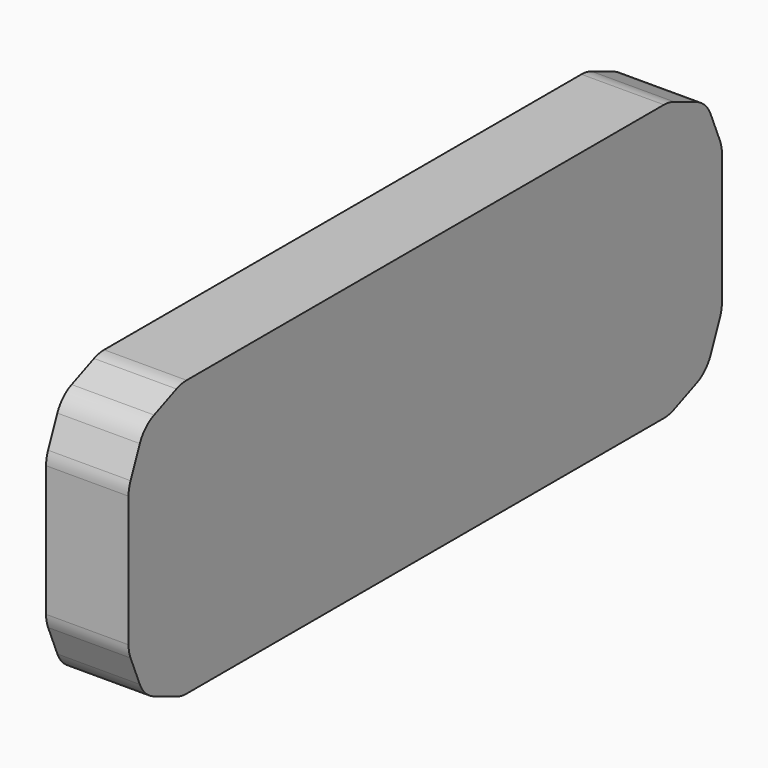
from build123d import *

# Parameters (mm, degrees)
F0_W        = 114.2217256129
F0_H        = 42.490478605
F1_DEPTH    = 12.7
F2_W        = 93.6551205814
F2_H        = 25.7396511734
F3_DEPTH    = 2.54
F4_R        = 5.08
F5_SIZE     = 5.08
F6_T1_DEPTH = 39.0415311919
F7_R        = 5.08


# Not quite as in the source:
# - a fillet or chamfer that OpenCascade refuses, or shapes differently, is made with other operations: its cross-section is extruded or revolved along the edge and cut away or added


with BuildPart() as f1:
    # F0 (on Right) → F1 (new body)
    with BuildSketch(Plane.YZ):
        with Locations((10.7826646417, 2.6869159192)):
            Rectangle(F0_W, F0_H)
    extrude(amount=F1_DEPTH)

    # F2 (on face) → F3 (join)
    with BuildSketch(Plane(origin=(0, 0, 0), x_dir=(0, -1, 0), z_dir=(-1, 0, 0))):
        with Locations((-10.6990095228, 3.1011626124)):
            Rectangle(F2_W, F2_H)
    extrude(amount=F3_DEPTH)

    # F4
    f4_edges = [f1.edges().sort_by_distance(p)[0] for p in [
        (-1.27, 57.52657, 15.970988),
        (-1.27, 57.52657, -9.768663),
        (-1.27, -36.128551, -9.768663),
        (-1.27, -36.128551, 15.970988),
    ]]
    fillet(f4_edges, radius=F4_R)

    # F5
    f5_edges = [f1.edges().sort_by_distance(p)[0] for p in [
        (6.35, 67.893527, 23.932155),
        (6.35, -46.328198, 23.932155),
        (6.35, 67.893527, -18.558323),
        (6.35, -46.328198, -18.558323),
    ]]
    chamfer(f5_edges, length=F5_SIZE)

    # F6: chamfer of 5.08 on 8 edges, made by hand

    # F6_s2 → F6_t1 (cut)
    with BuildSketch(Plane.YZ.offset(-13.170765596)):
        Polygon((64.3014249997, 22.4442576701), (67.8935274482, 13.7721552217), (67.8935274482, 18.8521552217), align=None)
        Polygon((57.7335274482, 23.9321552217), (66.4056298966, 20.3400527733), (62.8135274482, 23.9321552217), align=None)
        Polygon((66.4056298966, -14.9662209349), (57.7335274482, -18.5583233833), (62.8135274482, -18.5583233833), align=None)
        Polygon((67.8935274482, -8.3983233833), (64.3014249997, -17.0704258318), (67.8935274482, -13.4783233833), align=None)
        Polygon((-44.8403006131, -14.9662209349), (-36.1681981647, -18.5583233833), (-41.2481981647, -18.5583233833), align=None)
        Polygon((-46.3281981647, -8.3983233833), (-42.7360957163, -17.0704258318), (-46.3281981647, -13.4783233833), align=None)
        Polygon((-42.7360957163, 22.4442576701), (-46.3281981647, 13.7721552217), (-46.3281981647, 18.8521552217), align=None)
        Polygon((-36.1681981647, 23.9321552217), (-44.8403006131, 20.3400527733), (-41.2481981647, 23.9321552217), align=None)
    extrude(amount=F6_T1_DEPTH, mode=Mode.SUBTRACT)

    # F7
    f7_edges = [f1.edges().sort_by_distance(p)[0] for p in [
        (6.35, -43.352403, -15.582528),
        (6.35, -46.328198, -8.398323),
        (6.35, -36.168198, -18.558323),
        (6.35, -46.328198, 13.772155),
        (6.35, -43.352403, 20.95636),
        (6.35, -36.168198, 23.932155),
        (6.35, 57.733527, 23.932155),
        (6.35, 64.917732, 20.95636),
        (6.35, 67.893527, 13.772155),
        (6.35, 67.893527, -8.398323),
        (6.35, 64.917732, -15.582528),
        (6.35, 57.733527, -18.558323),
    ]]
    fillet(f7_edges, radius=F7_R)


solid = f1.part
